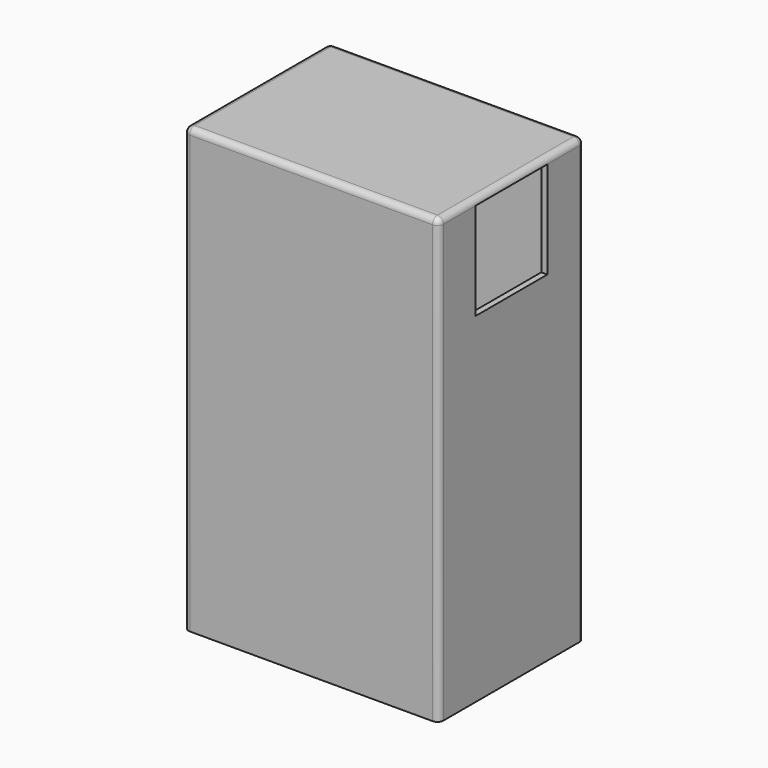
from build123d import *

# Parameters (mm, degrees)
F0_W      = 205
F0_H      = 360
F1_DEPTH  = 5
F2_W      = 150
F2_H      = 360
F3_DEPTH  = 5
F4_W      = 205
F4_H      = 360
F5_DEPTH  = 5
F6_W      = 205
F6_H      = 140
F7_DEPTH  = 5
F9_DEPTH  = 5
F10_R     = 5
F11_R     = 4.99999
F12_R     = 4.99999
F13_R     = 4.99999
F14_W     = 200
F14_H     = 140
F15_DEPTH = 110


# Not quite as in the source:
# - a fillet or chamfer is up to 0.001 mm smaller than in the source, because OpenCascade refuses the exact size


with BuildPart() as f1:
    # F0 (on Front) → F1 (new body)
    with BuildSketch(Plane.XZ):
        with Locations((102.5, 180)):
            Rectangle(F0_W, F0_H)
    extrude(amount=F1_DEPTH)

    # F2 (on face) → F3 (join)
    with BuildSketch(Plane(origin=(0, 0, 0), x_dir=(0, -1, 0), z_dir=(-1, 0, 0))):
        with Locations((-70, 180)):
            Rectangle(F2_W, F2_H)
    extrude(amount=F3_DEPTH)

    # F4 (on face) → F5 (join)
    with BuildSketch(Plane(origin=(0, 145, 0), x_dir=(-1, 0, 0), z_dir=(0, 1, 0))):
        with Locations((-102.5, 180)):
            Rectangle(F4_W, F4_H)
    extrude(amount=-F5_DEPTH)

    # F6 (on face) → F7 (join)
    with BuildSketch(Plane.XY.offset(360)):
        Polygon((-5, 145), (-5, -5), (205, -5), (205, 0), (0, 0), (0, 140), (205, 140), (205, 145), align=None)
        with Locations((102.5, 70)):
            Rectangle(F6_W, F6_H)
    extrude(amount=F7_DEPTH)

    # F10
    f10_edges = [f1.edges().sort_by_distance(p)[0] for p in [
        (205, -5, 182.5),
    ]]
    fillet(f10_edges, radius=F10_R)

    # F11 (radius 5 in the source; OpenCascade refuses exactly that, so slightly less here)
    f11_edges = [f1.edges().sort_by_distance(p)[0] for p in [
        (205, 72.5, 365),
    ]]
    fillet(f11_edges, radius=F11_R)

    # F12 (radius 5 in the source; OpenCascade refuses exactly that, so slightly less here)
    f12_edges = [f1.edges().sort_by_distance(p)[0] for p in [
        (205, 145, 180.000005),
    ]]
    fillet(f12_edges, radius=F12_R)

    # F13 (radius 5 in the source; OpenCascade refuses exactly that, so slightly less here)
    f13_edges = [f1.edges().sort_by_distance(p)[0] for p in [
        (-5, 70, 365),
    ]]
    fillet(f13_edges, radius=F13_R)


with BuildPart() as f9:
    # F8 (on face) → F9 (new body)
    with BuildSketch(Plane.YZ.offset(205)):
        Polygon((33, 280), (33, 360), (0, 360), (0, 0), (140, 0), (140, 360), (107, 360), (107, 280), align=None)
    extrude(amount=-F9_DEPTH)


with BuildPart() as f15:
    # F14 (on Top) → F15 (new body)
    with BuildSketch(Plane.XY):
        with Locations((100, 70)):
            Rectangle(F14_W, F14_H)
    extrude(amount=F15_DEPTH)


solid = Compound([f1.part, f9.part, f15.part])
